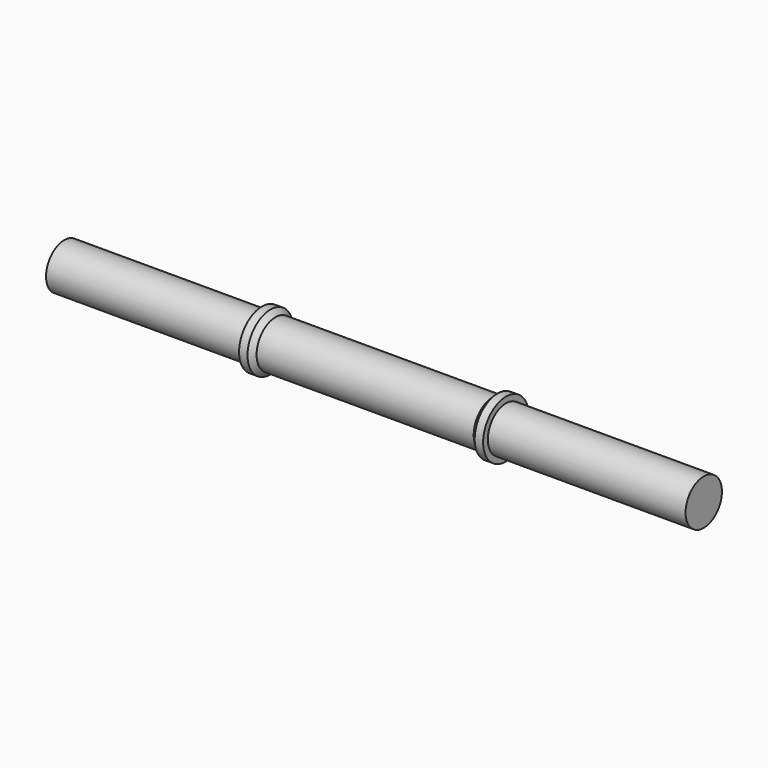
from build123d import *

# Parameters (mm, degrees)
F0_R     = 13.5
F1_DEPTH = 190
F2_R     = 17
F3_DEPTH = 72.5
F4_R     = 17.5
F4_R_2   = 14
F5_DEPTH = 67.5
F6_SIZE  = 2.99999


# Not quite as in the source:
# - a fillet or chamfer is up to 0.001 mm smaller than in the source, because OpenCascade refuses the exact size


with BuildPart() as f1:
    # F0 (on Right) → F1 (new body, symmetric)
    with BuildSketch(Plane.YZ):
        Circle(F0_R)
    extrude(amount=F1_DEPTH, both=True)

    # F2 (on Right) → F3 (join, symmetric)
    with BuildSketch(Plane.YZ):
        Circle(F2_R)
    extrude(amount=F3_DEPTH, both=True)

    # F4 (on Right) → F5 (cut, symmetric)
    with BuildSketch(Plane.YZ):
        Circle(F4_R)
        Circle(F4_R_2, mode=Mode.SUBTRACT)
    extrude(amount=F5_DEPTH, both=True, mode=Mode.SUBTRACT)

    # F6 (size 3 in the source; OpenCascade refuses exactly that, so slightly less here)
    f6_edges = [f1.edges().sort_by_distance(p)[0] for p in [
        (-67.5, -14, 0),
        (67.5, -14, 0),
    ]]
    chamfer(f6_edges, length=F6_SIZE)


solid = f1.part
